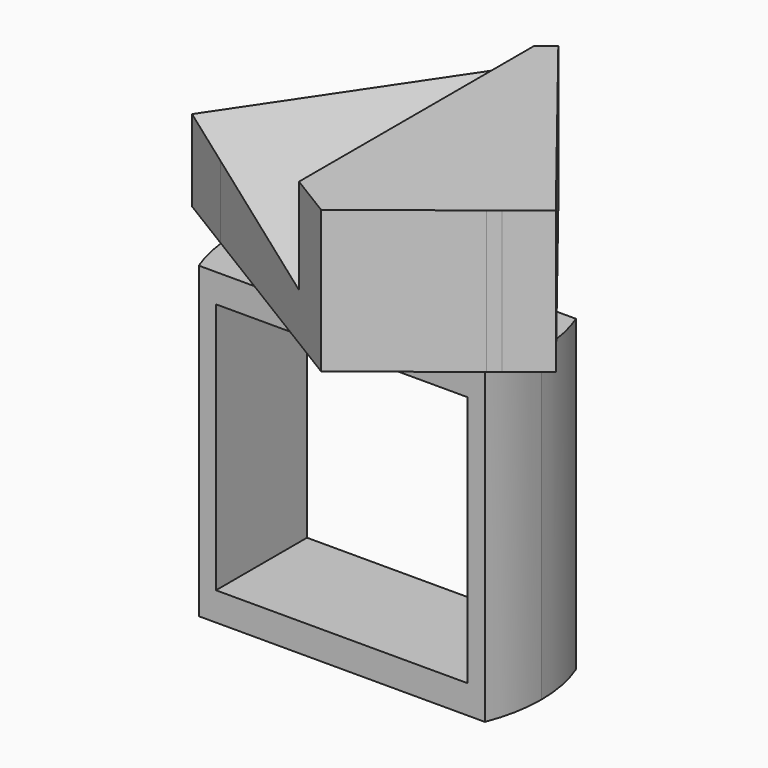
from build123d import *

# Parameters (mm, degrees)
F1_DEPTH      = 4
F1_DEPTH_BACK = 4
F3_DEPTH      = 10
F5_DEPTH      = 25
F7_DEPTH      = 21.7


with BuildPart() as f1:
    # F0 (on Front) → F1 (new body, two sides)
    with BuildSketch(Plane.XZ) as f1_sk:
        Polygon((-10.85, 10.85), (-10.85, 0), (-10.85, -10.85), (0, -10.85), (10.85, -10.85), (10.85, 0), (10.85, 10.85), (0, 10.85), align=None)
        Polygon((8.85, 8.85), (8.85, 0), (8.85, -8.85), (0, -8.85), (-8.85, -8.85), (-8.85, 0), (-8.85, 8.85), (0, 8.85), align=None, mode=Mode.SUBTRACT)
    extrude(amount=F1_DEPTH)
    extrude(f1_sk.sketch, amount=-F1_DEPTH_BACK)

    # F2 (on face) → F3 (join)
    with BuildSketch(Plane.XY.offset(10.85)):
        Polygon((-14.7346977867, 1.2544146994), (-10.85, -1.1231439692), (-10.85, 4), (8.7051686149, 4), (1.0543529996, 13.7034736867), align=None)
        Polygon((-6.1494992707, -4), (10.1865680069, -4), (10.85, -3.4769094021), (10.85, 1.2797259855), (8.7051686149, 4), (-10.85, 4), (-10.85, -1.1231439692), align=None)
        Polygon((-6.1494992707, -4), (3.047517268, -9.6288667992), (10.1865680069, -4), align=None)
        Polygon((10.85, 1.2797259855), (10.85, -3.4769094021), (13.1626902148, -1.6534421593), align=None)
    extrude(amount=F3_DEPTH)

    # F4 (on Right) → F5 (cut)
    with BuildSketch(Plane.YZ):
        Polygon((-36.6991721094, 6.3178054057), (17.9703272879, 21.0884753615), (-36.6991721094, 33.6725451052), align=None)
    extrude(amount=-F5_DEPTH, mode=Mode.SUBTRACT)

    # F6 (on face) → F7 (cut)
    with BuildSketch(Plane(origin=(0, 0, -10.85), x_dir=(1, 0, 0), z_dir=(0, 0, -1))):
        with BuildLine():
            Line((13.9217844345, 4.8126999282), (9.694906495, 4.8126999282))
            ThreePointArc((9.694906495, 4.8126999282), (9.8845588749, 4.4100780486), (10.0574993187, 4))
            Line((10.0574993187, 4), (10.85, 4))
            Line((10.85, 4), (10.85, -4))
            Line((10.85, -4), (10.0574993187, -4))
            ThreePointArc((10.0574993187, -4), (9.8311449192, -4.52790041), (9.5771050518, -5.0430498086))
            Line((9.5771050518, -5.0430498086), (13.9217844345, -5.0430498086))
            Line((13.9217844345, -5.0430498086), (13.9217844345, 4.8126999282))
        make_face()
        with BuildLine():
            Line((10.85, 4), (10.0574993187, 4))
            ThreePointArc((10.0574993187, 4), (10.6304521223, 2.0363644618), (10.8237374574, 0))
            ThreePointArc((10.8237374574, 0), (10.6304521223, -2.0363644618), (10.0574993187, -4))
            Line((10.0574993187, -4), (10.85, -4))
            Line((10.85, -4), (10.85, 4))
        make_face()
        with BuildLine():
            ThreePointArc((-10.0574993187, -4), (-10.8237374574, 0), (-10.0574993187, 4))
            Line((-10.0574993187, 4), (-10.85, 4))
            Line((-10.85, 4), (-10.85, -4))
            Line((-10.85, -4), (-10.0574993187, -4))
        make_face()
    extrude(amount=-F7_DEPTH, mode=Mode.SUBTRACT)


solid = f1.part
